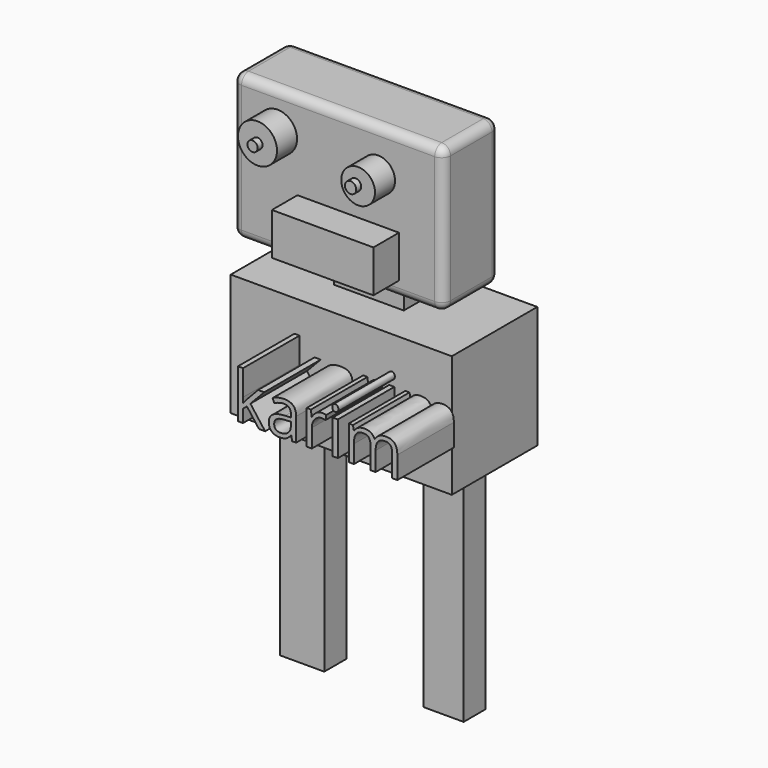
from build123d import *

# Parameters (mm, degrees)
F0_W          = 119.3729555234
F0_H          = 82.19993487
F1_DEPTH      = 39.3
F2_R          = 5
F3_R          = 9.5655435412
F3_R_2        = 11.0513986672
F4_DEPTH      = 14.2
F5_R          = 2.8930498294
F5_R_2        = 3.2214124145
F6_DEPTH      = 3.5
F7_W          = 57.4763091281
F7_H          = 23.8862577826
F8_DEPTH      = 18.1
F9_W          = 39.5616106689
F9_H          = 11.3832950592
F10_DEPTH     = 17.6
F11_W         = 125.2152733505
F11_H         = 60.5123713613
F11_W_2       = 39.5616106689
F11_H_2       = 11.3832950592
F12_DEPTH     = 69.1
F13_W         = 25.1925289631
F13_H         = 15.6753556803
F14_DEPTH     = 126.5
F15_TEXT_SIZE = 36.0421525935
F16_DEPTH     = 40


# Not quite as in the source:
# - Text() gives the source's letters only with a copy of the font that has no kerning and outlines rounded to 1/6400 em; it was checked with that copy


with BuildPart() as f1:
    # F0 (on Front) → F1 (new body)
    with BuildSketch(Plane.XZ):
        with Locations((-46.121370513, 8.3900820464)):
            Rectangle(F0_W, F0_H)
    extrude(amount=F1_DEPTH)

    # F2
    f2_edges = [f1.edges().sort_by_distance(p)[0] for p in [
        (-46.121371, -39.3, 49.490049),
        (-105.807848, -39.3, 8.390082),
        (13.565107, -39.3, 8.390082),
        (-46.121371, -39.3, -32.709885),
        (-46.121371, 0, 49.490049),
        (13.565107, 0, 8.390082),
        (-105.807848, 0, 8.390082),
        (-105.807848, -19.65, -32.709885),
        (-105.807848, -19.65, 49.490049),
        (13.565107, -19.65, 49.490049),
        (13.565107, -19.65, -32.709885),
        (-46.121371, 0, -32.709885),
    ]]
    fillet(f2_edges, radius=F2_R)

    # F3 (on face) → F4 (join)
    with BuildSketch(Plane.XZ.offset(39.3)):
        with Locations((-23.447688669, 25.128915906)):
            Circle(F3_R)
        with Locations((-80.438092351, 27.9393587261)):
            Circle(F3_R_2)
    extrude(amount=F4_DEPTH)

    # F5 (on face) → F6 (join)
    with BuildSketch(Plane.XZ.offset(53.5)):
        with Locations((-80.438092351, 27.9393587261)):
            Circle(F5_R)
        with Locations((-24.9211024493, 25.3791492432)):
            Circle(F5_R_2)
    extrude(amount=F6_DEPTH)

    # F7 (on face) → F8 (join)
    with BuildSketch(Plane.XZ.offset(39.3)):
        with Locations((-40.409849491, -11.9431288913)):
            Rectangle(F7_W, F7_H)
    extrude(amount=F8_DEPTH)

    # F9 (on face) → F10 (join)
    with BuildSketch(Plane(origin=(0, 0, -32.7098853886), x_dir=(1, 0, 0), z_dir=(0, 0, -1))):
        with Locations((-43.5822401196, 15.0222163647)):
            Rectangle(F9_W, F9_H)
    extrude(amount=F10_DEPTH)


with BuildPart() as f12:
    # F11 (on face) → F12 (new body)
    with BuildSketch(Plane(origin=(0, 0, -50.3098853886), x_dir=(1, 0, 0), z_dir=(0, 0, -1))):
        with Locations((-42.4658302218, 11.3985091448)):
            Rectangle(F11_W, F11_H)
        with Locations((-43.5822401196, 15.0222163647)):
            Rectangle(F11_W_2, F11_H_2, mode=Mode.SUBTRACT)
    extrude(amount=F12_DEPTH)

    # F13 (on face) → F14 (join)
    with BuildSketch(Plane(origin=(0, 0, -119.4098853886), x_dir=(1, 0, 0), z_dir=(0, 0, -1))):
        with Locations((-82.4907124043, 11.5699055605)):
            Rectangle(F13_W, F13_H)
        Polygon((8.2957223058, 18.4745267034), (-14.47086595, 18.4745267034), (-14.47086595, 2.9857822228), (-11.1118610948, 2.9857822228), (8.2957223058, 2.9857822228), align=None)
    extrude(amount=F14_DEPTH)

    # F15 (on face) → F16 (join)
    with BuildSketch(Plane.XZ.offset(41.6546948254)):
        with Locations((-72.0954686403, -95.4358428717)):
            Text('karim', F15_TEXT_SIZE, font='Open Sans', text_align=(TextAlign.LEFT, TextAlign.BOTTOM))
    extrude(amount=F16_DEPTH)


solid = Compound([f1.part, f12.part])
